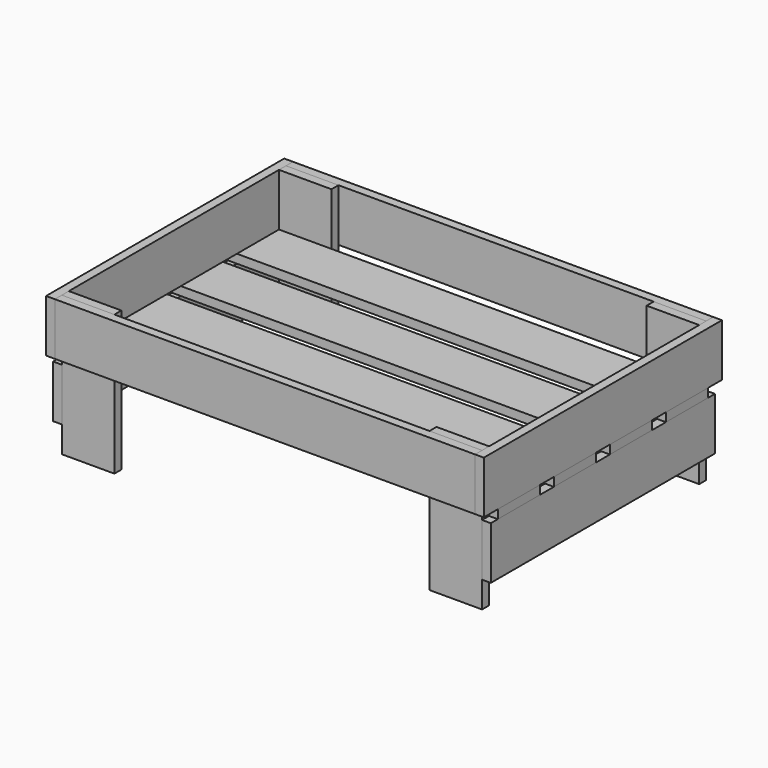
from build123d import *

# Parameters (mm, degrees)
F1_DEPTH  = 75
F0_W      = 1200
F0_H      = 25
F2_DEPTH  = 75
F3_W      = 150
F3_H      = 250
F3_H_2    = 150
F4_DEPTH  = 25
F5_START  = 750
F4_FACE_W = 150
F4_FACE_H = 400
F5_DEPTH  = 25
F6_W      = 1225
F6_H      = 150
F6_W_2    = 25
F7_DEPTH  = 25
F8_W      = 25
F8_H      = 150
F8_W_2    = 775
F9_DEPTH  = 25
F10_START = -1200
F10_DEPTH = 25
F11_DEPTH = 25


# Not quite as in the source:
# - a feature names something its author has since deleted; it is built from what else it names


with BuildPart() as f1:
    # F0 (on Top) → F1 (new body, symmetric)
    with BuildSketch(Plane.XY):
        Polygon((-611.2673640251, -401.8448650837), (-611.2673640251, 398.1551349163), (-611.2673640251, 423.1551349163), (-636.2673640251, 423.1551349163), (-636.2673640251, -426.8448650837), (-611.2673640251, -426.8448650837), align=None)
    extrude(amount=F1_DEPTH, both=True)


with BuildPart() as f1b:
    # F0 (on Top) → F1, piece 2 (new body, symmetric)
    with BuildSketch(Plane.XY):
        Polygon((588.7326359749, 423.1551349163), (588.7326359749, 398.1551349163), (588.7326359749, -401.8448650837), (588.7326359749, -426.8448650837), (613.7326359749, -426.8448650837), (613.7326359749, 423.1551349163), align=None)
    extrude(amount=F1_DEPTH, both=True)


with BuildPart() as f2:
    # F0 (on Top) → F2 (new body, symmetric)
    with BuildSketch(Plane.XY):
        with Locations((-11.2673640251, 410.6551349163)):
            Rectangle(F0_W, F0_H)
    extrude(amount=F2_DEPTH, both=True)


with BuildPart() as f2b:
    # F0 (on Top) → F2, piece 2 (new body, symmetric)
    with BuildSketch(Plane.XY):
        with Locations((-11.2673640251, -414.3448650837)):
            Rectangle(F0_W, F0_H)
    extrude(amount=F2_DEPTH, both=True)


with BuildPart() as f4:
    # F3 (on face) → F4 (new body)
    with BuildSketch(Plane.XZ.offset(-398.1551349163)):
        with Locations((513.7326359749, -200)):
            Rectangle(F3_W, F3_H)
        with Locations((513.7326359749, 0)):
            Rectangle(F3_W, F3_H_2)
    extrude(amount=F4_DEPTH)


with BuildPart() as f4b:
    # F3 (on face) → F4, piece 2 (new body)
    with BuildSketch(Plane.XZ.offset(-398.1551349163)):
        with Locations((-536.2673640251, 0)):
            Rectangle(F3_W, F3_H_2)
        with Locations((-536.2673640251, -200)):
            Rectangle(F3_W, F3_H)
    extrude(amount=F4_DEPTH)


with BuildPart() as f5:
    # F4_face (on face) → F5 (new body)
    with BuildSketch(Plane(origin=(-536.2673640251, 373.1551349163, -125), x_dir=(1, 0, 0), z_dir=(0, -1, 0)).offset(F5_START)):
        Rectangle(F4_FACE_W, F4_FACE_H)
    extrude(amount=F5_DEPTH)


with BuildPart() as f5b:
    # F4_face (on face) → F5, piece 2 (new body)
    with BuildSketch(Plane(origin=(-536.2673640251, 373.1551349163, -125), x_dir=(1, 0, 0), z_dir=(0, -1, 0)).offset(F5_START)):
        with Locations((1050, 0)):
            Rectangle(F4_FACE_W, F4_FACE_H)
    extrude(amount=F5_DEPTH)


with BuildPart() as f7:
    # F6 (on face) → F7 (new body)
    with BuildSketch(Plane(origin=(0, 0, -75), x_dir=(1, 0, 0), z_dir=(0, 0, -1))):
        with Locations((1.2326359749, -298.1551349163)):
            Rectangle(F6_W, F6_H)
        with Locations((-623.7673640251, -298.1551349163)):
            Rectangle(F6_W_2, F6_H)
    extrude(amount=F7_DEPTH)


with BuildPart() as f7b:
    # F6 (on face) → F7, piece 2 (new body)
    with BuildSketch(Plane(origin=(0, 0, -75), x_dir=(1, 0, 0), z_dir=(0, 0, -1))):
        with Locations((-623.7673640251, 301.8448650837)):
            Rectangle(F6_W_2, F6_H)
        with Locations((1.2326359749, 301.8448650837)):
            Rectangle(F6_W, F6_H)
    extrude(amount=F7_DEPTH)


with BuildPart() as f9:
    # F8 (on face) → F9 (new body)
    with BuildSketch(Plane(origin=(-611.2673640251, 0, 0), x_dir=(0, -1, 0), z_dir=(-1, 0, 0))):
        with Locations((-385.6551349163, -175)):
            Rectangle(F8_W, F8_H)
        with Locations((14.3448650837, -175)):
            Rectangle(F8_W_2, F8_H)
    extrude(amount=F9_DEPTH)


with BuildPart() as f10:
    # F8 (on face) → F10 (new body)
    with BuildSketch(Plane(origin=(-611.2673640251, 0, 0), x_dir=(0, -1, 0), z_dir=(-1, 0, 0)).offset(F10_START)):
        with Locations((14.3448650837, -175)):
            Rectangle(F8_W_2, F8_H)
        with Locations((-385.6551349163, -175)):
            Rectangle(F8_W, F8_H)
    extrude(amount=-F10_DEPTH)


with BuildPart() as f11:
    # F6 (on face) → F11 (new body)
    with BuildSketch(Plane(origin=(0, 0, -75), x_dir=(1, 0, 0), z_dir=(0, 0, -1))):
        with Locations((1.2326359749, 101.8448650837)):
            Rectangle(F6_W, F6_H)
        with Locations((-623.7673640251, 101.8448650837)):
            Rectangle(F6_W_2, F6_H)
    extrude(amount=F11_DEPTH)


with BuildPart() as f11b:
    # F6 (on face) → F11, piece 2 (new body)
    with BuildSketch(Plane(origin=(0, 0, -75), x_dir=(1, 0, 0), z_dir=(0, 0, -1))):
        with Locations((-623.7673640251, -98.1551349163)):
            Rectangle(F6_W_2, F6_H)
        with Locations((1.2326359749, -98.1551349163)):
            Rectangle(F6_W, F6_H)
    extrude(amount=F11_DEPTH)


solid = Compound([f1.part, f1b.part, f2.part, f2b.part, f4.part, f4b.part, f5.part, f5b.part, f7.part, f7b.part, f9.part, f10.part, f11.part, f11b.part])
